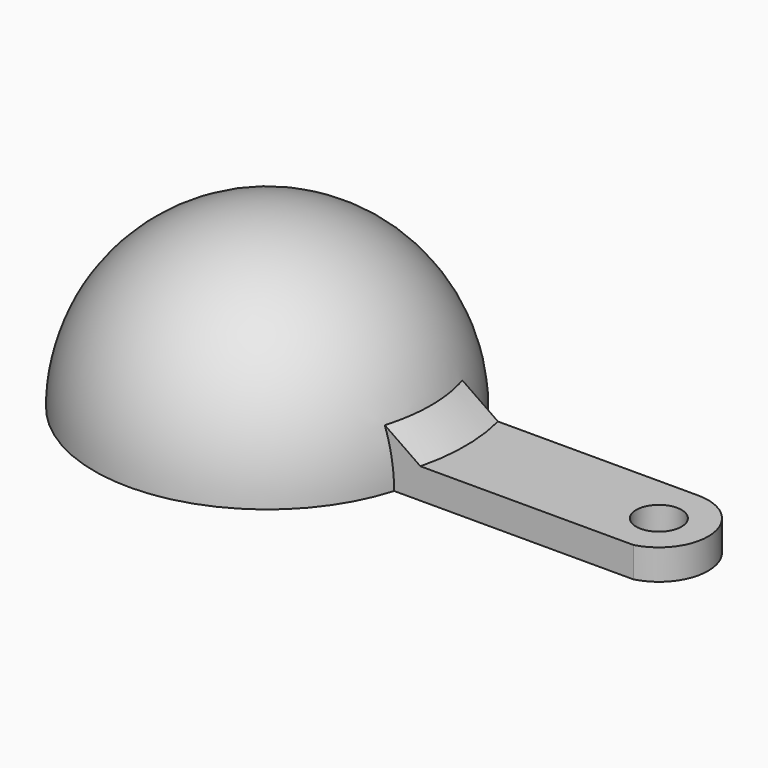
from build123d import *

# Parameters (mm, degrees)
F1_ANGLE    = 180
F2_R        = 3.75
F3_DEPTH    = 5
F4_T4_ANGLE = 81.9757587875


# Not quite as in the source:
# - a fillet or chamfer that OpenCascade refuses, or shapes differently, is made with other operations: its cross-section is extruded or revolved along the edge and cut away or added
# - a feature names something its author has since deleted; it is built from what else it names


with BuildPart() as f1:
    # F0 (on Top) → F1 (revolve)
    with BuildSketch(Plane.XY):
        with BuildLine():
            ThreePointArc((-26, 0), (0, 26), (26, 0))
            Line((26, 0), (28.5, 0))
            ThreePointArc((28.5, 0), (0, 28.5), (-28.5, 0))
            Line((-28.5, 0), (-26, 0))
        make_face()
    revolve(axis=Axis((0, 0, 0), (1, 0, 0)), revolution_arc=F1_ANGLE)

    # F2 (on Top) → F3 (join)
    with BuildSketch(Plane.XY):
        with BuildLine():
            Line((64.7386337537, 8), (24.7386337537, 8))
            ThreePointArc((24.7386337537, 8), (25.6827225737, 4.0494149209), (26, 0))
            ThreePointArc((26, 0), (25.6827225737, -4.0494149209), (24.7386337537, -8))
            Line((24.7386337537, -8), (66.83281573, -8))
            ThreePointArc((66.83281573, -8), (72.8068677326, 0.918971944), (64.7386337537, 8))
        make_face()
        with Locations((64.7386337537, -0.1370499422)):
            Circle(F2_R, mode=Mode.SUBTRACT)
    extrude(amount=F3_DEPTH)

    # F4: chamfer of 5 on 1 edges, made by hand


with BuildPart() as f4_tool2:
    # F4_s3 → F4_t4 (revolve)
    with BuildSketch(Plane(origin=(0, 0, 0), x_dir=(0, 0, 1), z_dir=(-0.6558993597, -0.754848349, 0))):
        with BuildLine():
            Line((4.8832304356, -32.8400371197), (9.1867076398, -26.8558845985))
            Line((9.1867076398, -26.8558845985), (9.1548832957, -26.761083696))
            ThreePointArc((9.1548832957, -26.761083696), (7.1037600734, -27.4972106371), (4.9824561404, -27.9595266557))
            Line((4.9824561404, -27.9595266557), (4.9, -28.0579756932))
            ThreePointArc((4.9, -28.0579756932), (4.9, -30.4490064064), (4.7832304356, -32.8400371197))
            Line((4.7832304356, -32.8400371197), (4.8832304356, -32.8400371197))
        make_face()
    revolve(axis=Axis((0, 0, 5), (0, 0, 1)), revolution_arc=F4_T4_ANGLE)

    split(bisect_by=Plane.XZ.offset(8), keep=Keep.BOTTOM)

    split(bisect_by=Plane.XZ.offset(-8), keep=Keep.TOP)


with BuildPart() as f1_1:
    add(f1.part)

    # F4_t1: union F4_tool2
    add(f4_tool2.part)


solid = f1_1.part
